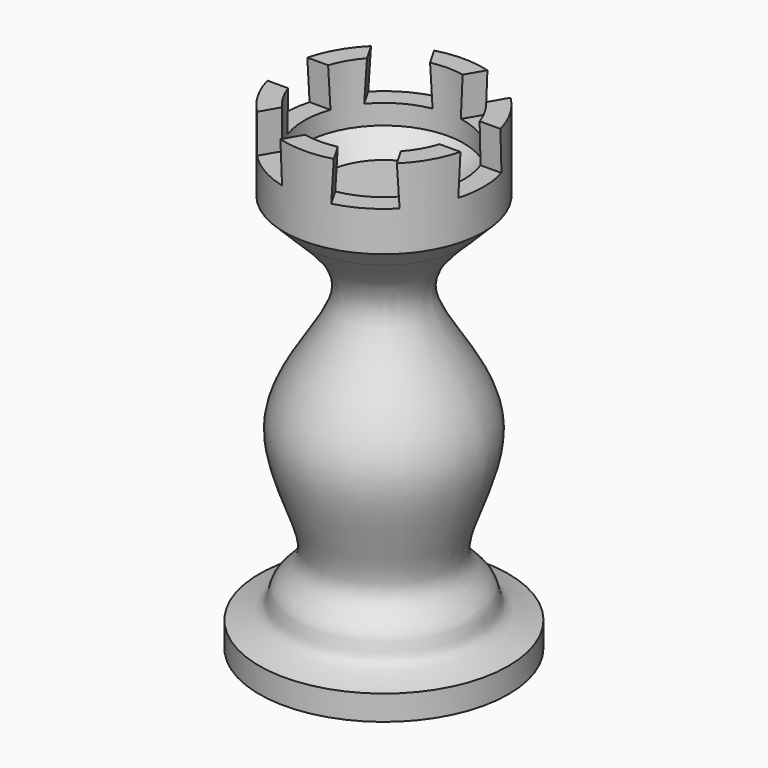
from build123d import *

# Parameters (mm, degrees)
F0_W            = 12.5
F0_H            = 2.5
F2_W            = 30
F2_H            = 5
F3_DEPTH        = 4
F3_TAPER        = -3
F3_COPIES_COUNT = 3
F3_COPIES_ANGLE = 120
F4_SIZE         = 2


# Not quite as in the source:
# - a pattern or mirror of a feature is missing from the dataset's text; its kind, count and spacing are read off the source's solid


with BuildPart() as f1:
    # F0 (on Front) → F1 (revolve)
    with BuildSketch(Plane.XZ):
        Polygon((10, 0), (8, 0), (8, -8), (0, -8), (0, -10), (8, -10), (10, -8), align=None)
        with BuildLine():
            Line((8, -10), (0, -10))
            Line((0, -10), (0, -45.5))
            Line((0, -45.5), (12.5, -45.5))
            add(Edge.make_bspline(
                [(8, -10), (5.9036325589, -11.9965153095), (1.0129290603, -16.5253438832), (13.2882333552, -27.2092652156), (4.5052088966, -39.5192070851), (9.2502525397, -41.9720056367), (8.9567015183, -44.5926383173), (11.3466967049, -45.1906230325), (12.5, -45.5)],
                knots=[0, 0, 0, 0, 0.1843856525, 0.4236571978, 0.6554974409, 0.7819959318, 0.8777293444, 1, 1, 1, 1], degree=3))
        make_face()
        with Locations((6.25, -46.75)):
            Rectangle(F0_W, F0_H)
    revolve(axis=Axis((0, 0, -24), (0, 0, -1)))

    # F2 (on face) → F3 (cut)
    with BuildSketch(Plane.XY):
        Rectangle(F2_W, F2_H)
    f3 = extrude(amount=-F3_DEPTH, taper=F3_TAPER, mode=Mode.SUBTRACT)

    # F3_copies: F3 ×3 about axis
    f3_copies_axis = Axis((0, 0, 0), (0, 0, 1))
    for i in range(1, F3_COPIES_COUNT):
        add(f3.rotate(f3_copies_axis, i * F3_COPIES_ANGLE / (F3_COPIES_COUNT - 1)), mode=Mode.SUBTRACT)

    # F4
    f4_edges = [f1.edges().sort_by_distance(p)[0] for p in [
        (-8, 0, -8),
    ]]
    chamfer(f4_edges, length=F4_SIZE)


solid = f1.part
